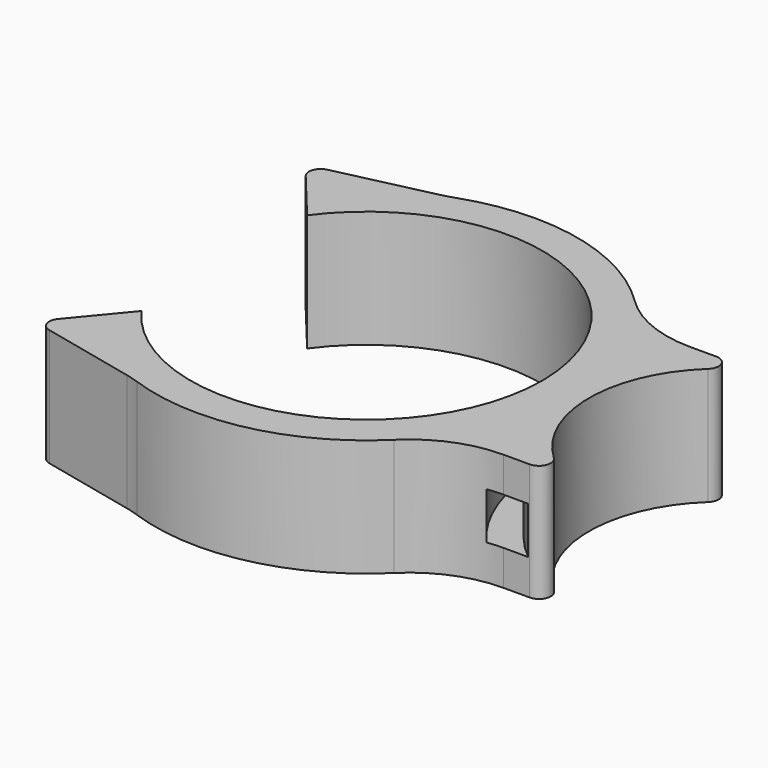
from build123d import *

# Parameters (mm, degrees)
F1_DEPTH = 10
F2_R     = 1
F3_R     = 10
F6_DEPTH = 4
F7_R     = 1


# Not quite as in the source:
# - ends of sketch curves that miss each other by under 0.0002 mm in the source are joined
# - a feature names something its author has since deleted; it is built from what else it names


with BuildPart() as f1:
    # F0 (on Top) → F1 (new body)
    with BuildSketch(Plane.XY):
        with BuildLine():
            ThreePointArc((-1.7962988307, -0.1596333839), (-12.2238763072, -14.2863823148), (-28.9155127569, -8.8376503509))
            Line((-28.9155127569, -8.8376503509), (-33.5614731624, -14.4524267481))
            Line((-33.5614731624, -14.4524267481), (-23.2513401401, -16.8024246609))
            ThreePointArc((-23.2513401401, -16.8024246609), (-11.3191539124, -17.1467252838), (-1.7954493794, -9.9498743711))
            Line((-1.7954493794, -9.9498743711), (8.2045506206, -9.9498743711))
            ThreePointArc((8.2045506206, -9.9498743711), (2.2045506206, 0), (8.2045506206, 9.9498743711))
            Line((8.2045506206, 9.9498743711), (-1.7954493794, 9.9498743711))
            ThreePointArc((-1.7954493794, 9.9498743711), (-11.3191539124, 17.1467252838), (-23.2513401401, 16.8024246609))
            Line((-23.2513401401, 16.8024246609), (-33.5614731624, 14.4524267481))
            Line((-33.5614731624, 14.4524267481), (-28.9155127569, 8.8376503509))
            ThreePointArc((-28.9155127569, 8.8376503509), (-12.3227425268, 14.3176427323), (-1.79993923, 0.3669814152))
            ThreePointArc((-1.79993923, 0.3669814152), (-1.7971307794, 0.2245866702), (-1.7956744539, 0.0821716783))
            Line((-1.7956744539, 0.0821716783), (-1.7954493794, 0.1693372455))
            Line((-1.7954493794, 0.1693372455), (-1.7954493794, 0.0497335093))
            ThreePointArc((-1.7954493794, 0.0497335093), (-1.795550035, -0.0549514122), (-1.7962988307, -0.1596333839))
        make_face()
        with BuildLine():
            Line((-1.7957105611, 0.0681883168), (-1.7962988307, -0.1596333839))
            ThreePointArc((-1.7962988307, -0.1596333839), (-1.795550035, -0.0549514122), (-1.7955318261, 0.049733236))
            Line((-1.7955318261, 0.049733236), (-1.7957105611, 0.0681883168))
        make_face()
        with BuildLine():
            Line((-1.7957105611, 0.0681883168), (-1.7954493794, 0.0497335093))
            ThreePointArc((-1.7954493794, 0.0497335093), (-1.7955943712, 0.0659524957), (-1.7956744539, 0.0821716783))
            Line((-1.7956744539, 0.0821716783), (-1.7957105611, 0.0681883168))
        make_face()
        with BuildLine():
            Line((-1.79993923, 0.3669814152), (-1.7957105611, 0.0681883168))
            Line((-1.7957105611, 0.0681883168), (-1.7956744539, 0.0821716783))
            ThreePointArc((-1.7956744539, 0.0821716783), (-1.7971307794, 0.2245866702), (-1.79993923, 0.3669814152))
        make_face()
    extrude(amount=F1_DEPTH)

    # F2
    f2_edges = [f1.edges().sort_by_distance(p)[0] for p in [
        (-33.561473, -14.452427, 5),
        (-33.561473, 14.452427, 5),
    ]]
    fillet(f2_edges, radius=F2_R)

    # F3
    f3_edges = [f1.edges().sort_by_distance(p)[0] for p in [
        (-1.795449, 9.949874, 5),
        (-1.795449, -9.949874, 5),
        (-23.25134, 16.802425, 5),
        (-23.25134, -16.802425, 5),
    ]]
    fillet(f3_edges, radius=F3_R)

    # F5 (on offset) → F6 (cut)
    with BuildSketch(Plane.XY.offset(7)):
        with BuildLine():
            ThreePointArc((11.5250723848, -12.6931975947), (0.3398769597, -1.8546317787), (7.9403583125, 11.740065307))
            Line((7.9403583125, 11.740065307), (3.2065206071, 11.740065307))
            ThreePointArc((3.2065206071, 11.740065307), (-2.2747136402, -0.7956794231), (4.4808682127, -12.6931975947))
            Line((4.4808682127, -12.6931975947), (11.5250723848, -12.6931975947))
        make_face()
    extrude(amount=-F6_DEPTH, mode=Mode.SUBTRACT)

    # F7
    f7_edges = [f1.edges().sort_by_distance(p)[0] for p in [
        (8.204551, 9.949874, 5),
        (8.204551, -9.949874, 5),
    ]]
    fillet(f7_edges, radius=F7_R)


solid = f1.part
